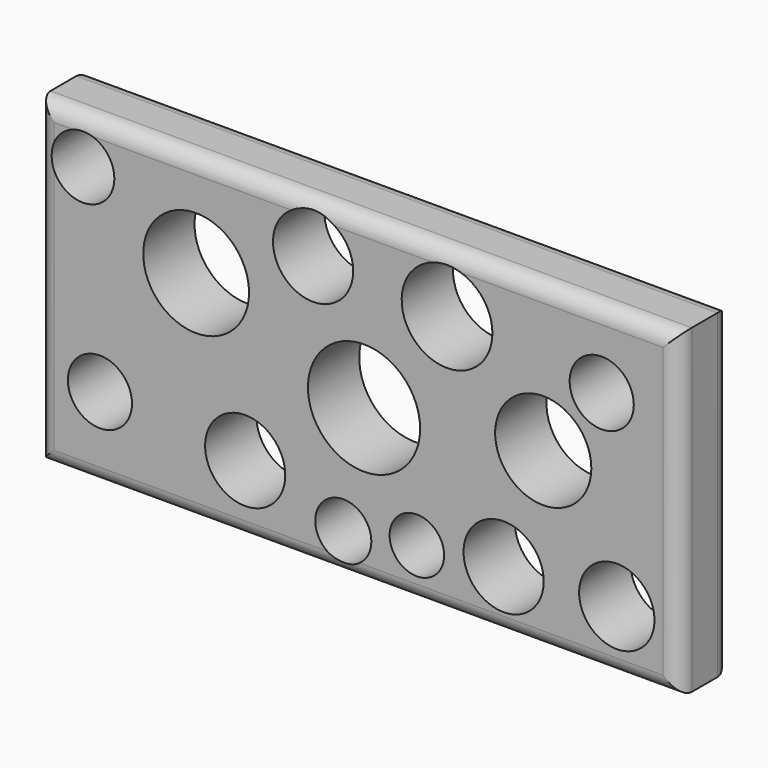
from build123d import *

# Parameters (mm, degrees)
F0_W        = 40
F0_H        = 20
F0_R        = 1.75
F0_R_2      = 2.5
F0_R_3      = 2
F0_R_4      = 1.7
F0_R_5      = 2.35
F0_R_6      = 3.5
F0_R_7      = 3.3
F0_R_8      = 1.9586185138
F0_R_9      = 3
F0_R_10     = 2.8292671529
F1_DEPTH    = 4
F2_T1_DEPTH = 25
F2_T3_DEPTH = 45


# Not quite as in the source:
# - a fillet or chamfer that OpenCascade refuses, or shapes differently, is made with other operations: its cross-section is extruded or revolved along the edge and cut away or added


with BuildPart() as f1:
    # F0 (on Front) → F1 (new body)
    with BuildSketch(Plane.XZ):
        with Locations((20, 10)):
            Rectangle(F0_W, F0_H)
        with Locations((19.0599078035, 2.4311765472)):
            Circle(F0_R, mode=Mode.SUBTRACT)
        with Locations((12.9404438354, 4.3140889982)):
            Circle(F0_R_2, mode=Mode.SUBTRACT)
        with Locations((3.878928961, 5.1378629939)):
            Circle(F0_R_3, mode=Mode.SUBTRACT)
        with Locations((23.6495067011, 3.1372687739)):
            Circle(F0_R_4, mode=Mode.SUBTRACT)
        with Locations((29.0628805159, 3.7256787709)):
            Circle(F0_R_2, mode=Mode.SUBTRACT)
        with Locations((36.1237967933, 3.8433607703)):
            Circle(F0_R_5, mode=Mode.SUBTRACT)
        with Locations((20.3544088753, 9.6097794314)):
            Circle(F0_R_6, mode=Mode.SUBTRACT)
        with Locations((9.8807118513, 13.6109674106)):
            Circle(F0_R_7, mode=Mode.SUBTRACT)
        with Locations((2.8197907362, 17.1414283137)):
            Circle(F0_R_8, mode=Mode.SUBTRACT)
        with Locations((17.1769958133, 16.9060624719)):
            Circle(F0_R_2, mode=Mode.SUBTRACT)
        with Locations((31.5342015816, 10.9042814246)):
            Circle(F0_R_9, mode=Mode.SUBTRACT)
        with Locations((25.5324186913, 16.3176533965)):
            Circle(F0_R_10, mode=Mode.SUBTRACT)
        with Locations((35.1823444841, 15.2585163235)):
            Circle(F0_R_3, mode=Mode.SUBTRACT)
    extrude(amount=F1_DEPTH)

    # F2: fillet of radius 1 on 8 edges, made by hand

    # F2_s2 → F2_t1 (cut)
    with BuildSketch(Plane.XY.offset(-2.5)):
        with BuildLine():
            ThreePointArc((0, -3), (0.2928932188, -3.7071067812), (1, -4))
            Line((1, -4), (0, -4))
            Line((0, -4), (0, -3))
        make_face()
        with BuildLine():
            ThreePointArc((40, -3), (39.7071067812, -3.7071067812), (39, -4))
            Line((39, -4), (40, -4))
            Line((40, -4), (40, -3))
        make_face()
        with BuildLine():
            ThreePointArc((0, -1), (0.2928932188, -0.2928932188), (1, 0))
            Line((1, 0), (0, 0))
            Line((0, 0), (0, -1))
        make_face()
        with BuildLine():
            ThreePointArc((40, -1), (39.7071067812, -0.2928932188), (39, 0))
            Line((39, 0), (40, 0))
            Line((40, 0), (40, -1))
        make_face()
    extrude(amount=F2_T1_DEPTH, mode=Mode.SUBTRACT)

    # F2_s4 → F2_t3 (cut)
    with BuildSketch(Plane.YZ.offset(-2.5)):
        with BuildLine():
            ThreePointArc((-3, 20), (-3.7071067812, 19.7071067812), (-4, 19))
            Line((-4, 19), (-4, 20))
            Line((-4, 20), (-3, 20))
        make_face()
        with BuildLine():
            ThreePointArc((-3, 0), (-3.7071067812, 0.2928932188), (-4, 1))
            Line((-4, 1), (-4, 0))
            Line((-4, 0), (-3, 0))
        make_face()
        with BuildLine():
            ThreePointArc((-1, 20), (-0.2928932188, 19.7071067812), (0, 19))
            Line((0, 19), (0, 20))
            Line((0, 20), (-1, 20))
        make_face()
        with BuildLine():
            ThreePointArc((-1, 0), (-0.2928932188, 0.2928932188), (0, 1))
            Line((0, 1), (0, 0))
            Line((0, 0), (-1, 0))
        make_face()
    extrude(amount=F2_T3_DEPTH, mode=Mode.SUBTRACT)


solid = f1.part
